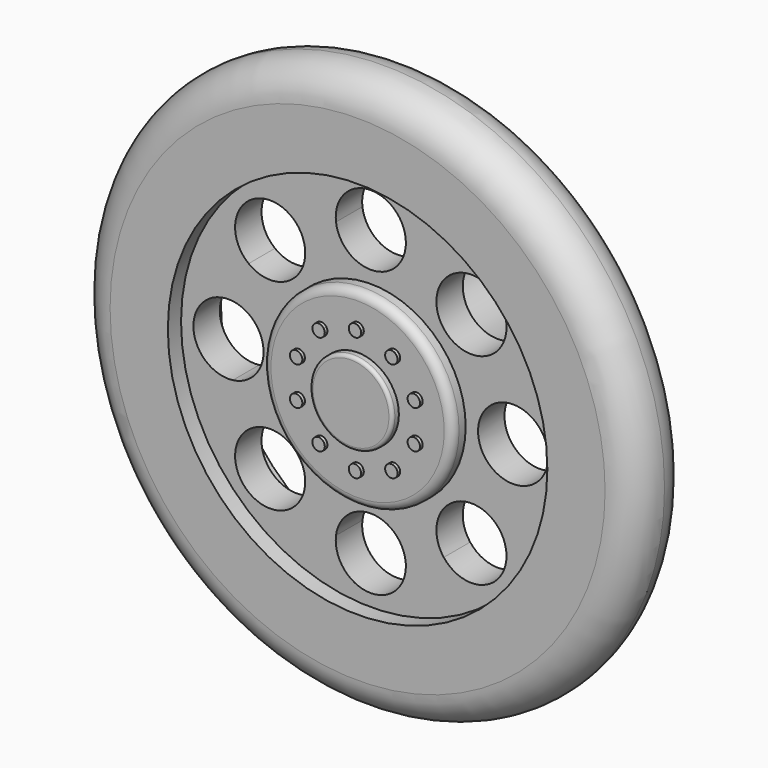
from build123d import *

# Parameters (mm, degrees)
F0_R      = 17
F1_DEPTH  = 4
F2_R      = 11.5
F3_DEPTH  = 1
F4_R      = 11.5
F5_DEPTH  = 1
F6_R      = 2
F7_R      = 1.99999
F8_R      = 2.5
F9_DEPTH  = 1.5
F10_R     = 5.75
F11_DEPTH = 1
F12_R     = 0.5
F13_R     = 0.2
F15_DEPTH = 25.4
F16_R     = 3
F16_R_2   = 2.25
F17_DEPTH = 7.5
F19_DEPTH = 0.2


# Not quite as in the source:
# - a fillet or chamfer is up to 0.001 mm smaller than in the source, because OpenCascade refuses the exact size


with BuildPart() as f1:
    # F0 (on Front) → F1 (new body)
    with BuildSketch(Plane.XZ):
        Circle(F0_R)
    extrude(amount=-F1_DEPTH)

    # F2 (on face) → F3 (cut)
    with BuildSketch(Plane.XZ):
        Circle(F2_R)
    extrude(amount=-F3_DEPTH, mode=Mode.SUBTRACT)

    # F4 (on face) → F5 (cut)
    with BuildSketch(Plane(origin=(0, 4, 0), x_dir=(-1, 0, 0), z_dir=(0, 1, 0))):
        Circle(F4_R)
    extrude(amount=-F5_DEPTH, mode=Mode.SUBTRACT)

    # F6
    f6_edges = [f1.edges().sort_by_distance(p)[0] for p in [
        (-17, 0, 0),
    ]]
    fillet(f6_edges, radius=F6_R)

    # F7 (radius 2 in the source; OpenCascade refuses exactly that, so slightly less here)
    f7_edges = [f1.edges().sort_by_distance(p)[0] for p in [
        (-17, 4, 0),
    ]]
    fillet(f7_edges, radius=F7_R)

    # F8 (on face) → F9 (join)
    with BuildSketch(Plane.XZ.offset(-1)):
        Circle(F8_R)
    extrude(amount=F9_DEPTH)

    # F10 (on face) → F11 (join)
    with BuildSketch(Plane.XZ.offset(-1)):
        Circle(F10_R)
    extrude(amount=F11_DEPTH)

    # F12
    f12_edges = [f1.edges().sort_by_distance(p)[0] for p in [
        (-5.75, 0, 0),
    ]]
    fillet(f12_edges, radius=F12_R)

    # F13
    f13_edges = [f1.edges().sort_by_distance(p)[0] for p in [
        (-2.5, -0.5, 0),
    ]]
    fillet(f13_edges, radius=F13_R)

    # F14 (on face) → F15 (cut)
    with BuildSketch(Plane.XZ.offset(-1)):
        with BuildLine():
            ThreePointArc((-2.1088145152, 8.3632246377), (0, 6.5), (2.1088145152, 8.3632246377))
            ThreePointArc((2.1088145152, 8.3632246377), (0, 8.625), (-2.1088145152, 8.3632246377))
        make_face()
        with BuildLine():
            ThreePointArc((-2.1088145152, 8.3632246377), (0, 8.625), (2.1088145152, 8.3632246377))
            ThreePointArc((2.1088145152, 8.3632246377), (2.120949769, 8.4938623717), (2.125, 8.625))
            ThreePointArc((2.125, 8.625), (-0.1311376283, 10.745949769), (-2.1088145152, 8.3632246377))
        make_face()
        with BuildLine():
            ThreePointArc((-3.9737959877, 6.0987959877), (-4.089109709, 6.7892929545), (-4.4225358099, 7.4048498979))
            ThreePointArc((-4.4225358099, 7.4048498979), (-6.0987959877, 6.0987959877), (-7.4048498979, 4.4225358099))
            ThreePointArc((-7.4048498979, 4.4225358099), (-5.1659882795, 4.1894781044), (-3.9737959877, 6.0987959877))
        make_face()
        with BuildLine():
            ThreePointArc((-7.4048498979, 4.4225358099), (-6.0987959877, 6.0987959877), (-4.4225358099, 7.4048498979))
            ThreePointArc((-4.4225358099, 7.4048498979), (-7.6013978978, 7.6013978978), (-7.4048498979, 4.4225358099))
        make_face()
        with BuildLine():
            ThreePointArc((-6.5, 0), (-7.0325337296, 1.4070096579), (-8.3632246377, 2.1088145152))
            ThreePointArc((-8.3632246377, 2.1088145152), (-8.625, 0), (-8.3632246377, -2.1088145152))
            ThreePointArc((-8.3632246377, -2.1088145152), (-7.0325337296, -1.4070096579), (-6.5, 0))
        make_face()
        with BuildLine():
            ThreePointArc((-8.3632246377, -2.1088145152), (-8.625, 0), (-8.3632246377, 2.1088145152))
            ThreePointArc((-8.3632246377, 2.1088145152), (-10.75, 0), (-8.3632246377, -2.1088145152))
        make_face()
        with BuildLine():
            ThreePointArc((-7.4048498979, -4.4225358099), (-7.6013978978, -7.6013978978), (-4.4225358099, -7.4048498979))
            ThreePointArc((-4.4225358099, -7.4048498979), (-6.0987959877, -6.0987959877), (-7.4048498979, -4.4225358099))
        make_face()
        with BuildLine():
            ThreePointArc((-7.4048498979, -4.4225358099), (-6.0987959877, -6.0987959877), (-4.4225358099, -7.4048498979))
            ThreePointArc((-4.4225358099, -7.4048498979), (-4.089109709, -6.7892929545), (-3.9737959877, -6.0987959877))
            ThreePointArc((-3.9737959877, -6.0987959877), (-5.1659882795, -4.1894781044), (-7.4048498979, -4.4225358099))
        make_face()
        with BuildLine():
            ThreePointArc((2.125, -8.625), (2.120949769, -8.4938623717), (2.1088145152, -8.3632246377))
            ThreePointArc((2.1088145152, -8.3632246377), (0, -8.625), (-2.1088145152, -8.3632246377))
            ThreePointArc((-2.1088145152, -8.3632246377), (-0.1311376283, -10.745949769), (2.125, -8.625))
        make_face()
        with BuildLine():
            ThreePointArc((-2.1088145152, -8.3632246377), (0, -8.625), (2.1088145152, -8.3632246377))
            ThreePointArc((2.1088145152, -8.3632246377), (0, -6.5), (-2.1088145152, -8.3632246377))
        make_face()
        with BuildLine():
            ThreePointArc((8.2237959877, -6.0987959877), (8.008113871, -5.1659882795), (7.4048498979, -4.4225358099))
            ThreePointArc((7.4048498979, -4.4225358099), (6.0987959877, -6.0987959877), (4.4225358099, -7.4048498979))
            ThreePointArc((4.4225358099, -7.4048498979), (6.7892929545, -8.1084822665), (8.2237959877, -6.0987959877))
        make_face()
        with BuildLine():
            ThreePointArc((4.4225358099, -7.4048498979), (6.0987959877, -6.0987959877), (7.4048498979, -4.4225358099))
            ThreePointArc((7.4048498979, -4.4225358099), (4.5961940777, -4.5961940777), (4.4225358099, -7.4048498979))
        make_face()
        with BuildLine():
            ThreePointArc((8.3632246377, -2.1088145152), (8.5593059736, -1.0625), (8.625, 0))
            ThreePointArc((8.625, 0), (8.5593059736, 1.0625), (8.3632246377, 2.1088145152))
            ThreePointArc((8.3632246377, 2.1088145152), (6.5, 0), (8.3632246377, -2.1088145152))
        make_face()
        with BuildLine():
            ThreePointArc((8.3632246377, 2.1088145152), (8.5593059736, 1.0625), (8.625, 0))
            ThreePointArc((8.625, 0), (8.5593059736, -1.0625), (8.3632246377, -2.1088145152))
            ThreePointArc((8.3632246377, -2.1088145152), (10.0320096579, -1.5924662704), (10.75, 0))
            ThreePointArc((10.75, 0), (10.0320096579, 1.5924662704), (8.3632246377, 2.1088145152))
        make_face()
        with BuildLine():
            ThreePointArc((4.4225358099, 7.4048498979), (6.0987959877, 6.0987959877), (7.4048498979, 4.4225358099))
            ThreePointArc((7.4048498979, 4.4225358099), (8.008113871, 5.1659882795), (8.2237959877, 6.0987959877))
            ThreePointArc((8.2237959877, 6.0987959877), (6.7892929545, 8.1084822665), (4.4225358099, 7.4048498979))
        make_face()
        with BuildLine():
            ThreePointArc((4.4225358099, 7.4048498979), (4.5961940777, 4.5961940777), (7.4048498979, 4.4225358099))
            ThreePointArc((7.4048498979, 4.4225358099), (6.0987959877, 6.0987959877), (4.4225358099, 7.4048498979))
        make_face()
    extrude(amount=-F15_DEPTH, mode=Mode.SUBTRACT)

    # F16 (on face) → F17 (join)
    with BuildSketch(Plane(origin=(0, 3, 0), x_dir=(-1, 0, 0), z_dir=(0, 1, 0))):
        Circle(F16_R)
        Circle(F16_R_2, mode=Mode.SUBTRACT)
    extrude(amount=F17_DEPTH)

    # F18 (on face) → F19 (join)
    with BuildSketch(Plane.XZ):
        with BuildLine():
            ThreePointArc((3.4328931959, 1.5092197672), (3.2098157425, 1.042932356), (3.664366057, 0.7968195534))
            ThreePointArc((3.664366057, 0.7968195534), (3.5664619361, 1.1588137289), (3.4328931959, 1.5092197672))
        make_face()
        with BuildLine():
            ThreePointArc((3.4328931959, 1.5092197672), (3.5664619361, 1.1588137289), (3.664366057, 0.7968195534))
            ThreePointArc((3.664366057, 0.7968195534), (3.8642362175, 0.9308762872), (3.9414619361, 1.1588137289))
            ThreePointArc((3.9414619361, 1.1588137289), (3.7792255637, 1.4676124316), (3.4328931959, 1.5092197672))
        make_face()
        with BuildLine():
            ThreePointArc((3.9414619361, -1.1588137289), (3.8642362175, -0.9308762872), (3.664366057, -0.7968195534))
            ThreePointArc((3.664366057, -0.7968195534), (3.5664619361, -1.1588137289), (3.4328931959, -1.5092197672))
            ThreePointArc((3.4328931959, -1.5092197672), (3.7792255637, -1.4676124316), (3.9414619361, -1.1588137289))
        make_face()
        with BuildLine():
            ThreePointArc((3.4328931959, -1.5092197672), (3.5664619361, -1.1588137289), (3.664366057, -0.7968195534))
            ThreePointArc((3.664366057, -0.7968195534), (3.2098157425, -1.042932356), (3.4328931959, -1.5092197672))
        make_face()
        with BuildLine():
            ThreePointArc((1.8901718138, 3.2387884331), (1.9837752265, 2.730432356), (2.4961756315, 2.7985008874))
            ThreePointArc((2.4961756315, 2.7985008874), (2.2041946961, 3.0338137289), (1.8901718138, 3.2387884331))
        make_face()
        with BuildLine():
            ThreePointArc((1.8901718138, 3.2387884331), (2.2041946961, 3.0338137289), (2.4961756315, 2.7985008874))
            ThreePointArc((2.4961756315, 2.7985008874), (2.5578314099, 2.9090496531), (2.5791946961, 3.0338137289))
            ThreePointArc((2.5791946961, 3.0338137289), (2.3111208835, 3.393246324), (1.8901718138, 3.2387884331))
        make_face()
        with BuildLine():
            ThreePointArc((2.5791946961, -3.0338137289), (2.5578314099, -2.9090496531), (2.4961756315, -2.7985008874))
            ThreePointArc((2.4961756315, -2.7985008874), (2.2041946961, -3.0338137289), (1.8901718138, -3.2387884331))
            ThreePointArc((1.8901718138, -3.2387884331), (2.3111208835, -3.393246324), (2.5791946961, -3.0338137289))
        make_face()
        with BuildLine():
            ThreePointArc((1.8901718138, -3.2387884331), (2.2041946961, -3.0338137289), (2.4961756315, -2.7985008874))
            ThreePointArc((2.4961756315, -2.7985008874), (1.9837752265, -2.730432356), (1.8901718138, -3.2387884331))
        make_face()
        with BuildLine():
            ThreePointArc((-0.3745309567, 3.73125), (0, 3.375), (0.3745309567, 3.73125))
            ThreePointArc((0.3745309567, 3.73125), (0, 3.75), (-0.3745309567, 3.73125))
        make_face()
        with BuildLine():
            ThreePointArc((-0.3745309567, 3.73125), (0, 3.75), (0.3745309567, 3.73125))
            ThreePointArc((0.3745309567, 3.73125), (0.3748827208, 3.7406220671), (0.375, 3.75))
            ThreePointArc((0.375, 3.75), (-0.0093779329, 4.1248827208), (-0.3745309567, 3.73125))
        make_face()
        with BuildLine():
            ThreePointArc((0.375, -3.75), (0.3748827208, -3.7406220671), (0.3745309567, -3.73125))
            ThreePointArc((0.3745309567, -3.73125), (0, -3.75), (-0.3745309567, -3.73125))
            ThreePointArc((-0.3745309567, -3.73125), (-0.0093779329, -4.1248827208), (0.375, -3.75))
        make_face()
        with BuildLine():
            ThreePointArc((-0.3745309567, -3.73125), (0, -3.75), (0.3745309567, -3.73125))
            ThreePointArc((0.3745309567, -3.73125), (0, -3.375), (-0.3745309567, -3.73125))
        make_face()
        with BuildLine():
            ThreePointArc((-1.8291946961, 3.0338137289), (-1.844762101, 3.1407399163), (-1.8901718138, 3.2387884331))
            ThreePointArc((-1.8901718138, 3.2387884331), (-2.2041946961, 3.0338137289), (-2.4961756315, 2.7985008874))
            ThreePointArc((-2.4961756315, 2.7985008874), (-2.0794306203, 2.6801770151), (-1.8291946961, 3.0338137289))
        make_face()
        with BuildLine():
            ThreePointArc((-2.4961756315, 2.7985008874), (-2.2041946961, 3.0338137289), (-1.8901718138, 3.2387884331))
            ThreePointArc((-1.8901718138, 3.2387884331), (-2.4246141657, 3.3371951018), (-2.4961756315, 2.7985008874))
        make_face()
        with BuildLine():
            ThreePointArc((-2.4961756315, -2.7985008874), (-2.4246141657, -3.3371951018), (-1.8901718138, -3.2387884331))
            ThreePointArc((-1.8901718138, -3.2387884331), (-2.2041946961, -3.0338137289), (-2.4961756315, -2.7985008874))
        make_face()
        with BuildLine():
            ThreePointArc((-2.4961756315, -2.7985008874), (-2.2041946961, -3.0338137289), (-1.8901718138, -3.2387884331))
            ThreePointArc((-1.8901718138, -3.2387884331), (-1.844762101, -3.1407399163), (-1.8291946961, -3.0338137289))
            ThreePointArc((-1.8291946961, -3.0338137289), (-2.0794306203, -2.6801770151), (-2.4961756315, -2.7985008874))
        make_face()
        with BuildLine():
            ThreePointArc((-3.1914619361, 1.1588137289), (-3.2576632334, 1.3715773565), (-3.4328931959, 1.5092197672))
            ThreePointArc((-3.4328931959, 1.5092197672), (-3.5664619361, 1.1588137289), (-3.664366057, 0.7968195534))
            ThreePointArc((-3.664366057, 0.7968195534), (-3.3385244944, 0.8610394475), (-3.1914619361, 1.1588137289))
        make_face()
        with BuildLine():
            ThreePointArc((-3.664366057, 0.7968195534), (-3.5664619361, 1.1588137289), (-3.4328931959, 1.5092197672))
            ThreePointArc((-3.4328931959, 1.5092197672), (-3.9231081297, 1.2746951018), (-3.664366057, 0.7968195534))
        make_face()
        with BuildLine():
            ThreePointArc((-3.664366057, -0.7968195534), (-3.9231081297, -1.2746951018), (-3.4328931959, -1.5092197672))
            ThreePointArc((-3.4328931959, -1.5092197672), (-3.5664619361, -1.1588137289), (-3.664366057, -0.7968195534))
        make_face()
        with BuildLine():
            ThreePointArc((-3.664366057, -0.7968195534), (-3.5664619361, -1.1588137289), (-3.4328931959, -1.5092197672))
            ThreePointArc((-3.4328931959, -1.5092197672), (-3.2576632334, -1.3715773565), (-3.1914619361, -1.1588137289))
            ThreePointArc((-3.1914619361, -1.1588137289), (-3.3385244944, -0.8610394475), (-3.664366057, -0.7968195534))
        make_face()
    extrude(amount=F19_DEPTH)


solid = f1.part
